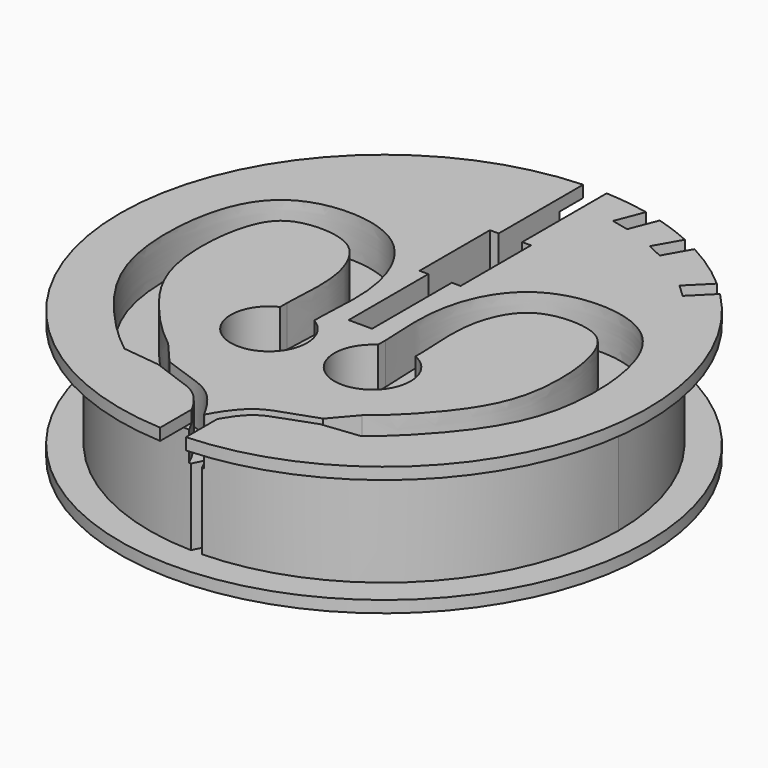
from build123d import *

# Parameters (mm, degrees)
F0_R           = 6.5
F1_DEPTH       = 22
F3_DEPTH       = 7
F5_DEPTH       = 6
F4_W           = 4
F4_H           = 17
F6_DEPTH       = 6
F7_DEPTH       = 9
F8_R           = 45
F8_R_2         = 40
F9_DEPTH       = 2
F10_START      = 20
F10_DEPTH      = 2
F11_DEPTH      = 4
F13_DEPTH      = 15
F13_DEPTH_BACK = 2
F14_W          = 3.2336955192
F14_H          = 3.9470121264
F15_DEPTH      = 2
F17_START      = 18
F17_DEPTH      = 4


# Not quite as in the source:
# - the dataset's text gives a spline's control points without its knots; the knots are read off the source's solid


with BuildPart() as f1:
    # F0 (on Top) → F1 (new body)
    with BuildSketch(Plane.XY):
        with BuildLine():
            ThreePointArc((0.9474656624, -39.9887772859), (28.6172904596, -27.9472840676), (40, 0))
            ThreePointArc((40, 0), (-27.9472840676, 28.6172904596), (-0.9474656624, -39.9887772859))
            add(Edge.make_bspline(
                [(0, -38.0722548049), (-0.3439047687, -38.7199985815), (-0.6597297626, -39.3669666276), (-0.9474656624, -39.9887772859)],
                knots=[0.8933636625, 0.8933636625, 0.8933636625, 0.8933636625, 1, 1, 1, 1], degree=3))
            add(Edge.make_bspline(
                [(0, -38.0722548049), (0.3439047687, -38.7199985815), (0.6597297626, -39.3669666276), (0.9474656624, -39.9887772859)],
                knots=[0.8933636625, 0.8933636625, 0.8933636625, 0.8933636625, 1, 1, 1, 1], degree=3))
        make_face()
        with Locations((-8.6927901772, -13.6614393054)):
            Circle(F0_R, mode=Mode.SUBTRACT)
        with Locations((8.9704493242, -13.6614393054)):
            Circle(F0_R, mode=Mode.SUBTRACT)
    extrude(amount=F1_DEPTH)

    # F2 (on face) → F3 (cut)
    with BuildSketch(Plane.XY.offset(22)):
        with BuildLine():
            Line((-11.4866509255, -6.2936628617), (-5.4897859509, -6.4875970689))
            add(Edge.make_bspline(
                [(-5.4897859509, -6.4875970689), (-5.4379960808, -4.8861423136), (-5.2594316262, -2.3960567313), (-5.21271863, 1.1661147071), (-5.3919407568, 3.966171195), (-5.9185254374, 6.8935002169), (-6.854038873, 9.8103742554), (-8.0244197776, 12.1448151724), (-9.2394760694, 13.8844575869), (-10.3025573556, 15.1020966662), (-11.5243351598, 16.2052705185), (-12.9191140784, 17.1606232553), (-14.3946005778, 17.9101133701), (-16.4368763853, 18.6735386839), (-19.0722321519, 19.2235783462), (-22.2281493374, 19.3375488673), (-24.7519752983, 19.0203587631), (-26.6553594717, 18.5206918318), (-28.4891702037, 17.8345146965), (-30.6169895374, 16.5861777721), (-32.3874729615, 14.8001880422), (-33.5420378244, 13.1039536454), (-34.2835644411, 11.7074846102), (-34.9043465841, 10.2008340024), (-35.5860681144, 8.0784891374), (-36.1962974623, 5.2321659425), (-36.5786674883, 1.6179124526), (-36.6190440844, -2.0722357876), (-36.3636264791, -5.1013980108), (-35.9747219859, -7.4398512499), (-35.4580158659, -9.6887320868), (-34.5932379657, -12.3018318431), (-33.2617334438, -15.1551375454), (-31.7045842952, -17.7556472269), (-30.2724053046, -19.7527908698), (-29.0788395713, -21.2722688411), (-27.8491903942, -22.7627774848), (-26.2467211141, -24.5683632891), (-23.5869366027, -27.2873636582), (-21.5286445413, -29.0857624272), (-20.1586929343, -30.1331636176)],
                knots=[0, 0, 0, 0, 0.0625, 0.09375, 0.125, 0.15625, 0.1875, 0.21875, 0.234375, 0.25, 0.265625, 0.28125, 0.296875, 0.3125, 0.34375, 0.375, 0.40625, 0.421875, 0.4375, 0.46875, 0.5, 0.515625, 0.53125, 0.546875, 0.5625, 0.59375, 0.625, 0.65625, 0.6875, 0.703125, 0.71875, 0.75, 0.78125, 0.8125, 0.84375, 0.859375, 0.875, 0.90625, 0.9375, 1, 1, 1, 1], degree=3))
            Line((-20.1586929343, -30.1331636176), (-16.5144508549, -25.3666659866))
            add(Edge.make_bspline(
                [(-11.4866509255, -6.2936628617), (-11.4582628575, -5.4158424255), (-11.3694789243, -3.707307233), (-11.2442598399, -1.2739253297), (-11.2217249783, 0.6576847954), (-11.2909792301, 2.1555003202), (-11.3951046961, 3.2596312313), (-11.5599404384, 4.3484374353), (-11.7949569978, 5.4365525911), (-12.100056325, 6.5030976742), (-12.5990453032, 7.8712270505), (-13.2319794554, 9.1203362077), (-13.9810727023, 10.1887494849), (-14.5951072186, 10.889894646), (-15.2595373513, 11.4865430576), (-15.97150147, 11.975035844), (-16.8044210088, 12.4016945204), (-18.0437162501, 12.8672967201), (-19.7854683017, 13.2380556024), (-21.6065908286, 13.3043531415), (-22.9949988463, 13.1866711855), (-23.9731162944, 13.0200835746), (-24.8514199077, 12.7876330323), (-25.8679172481, 12.4033835088), (-26.8953272178, 11.7912643881), (-27.7498799628, 10.9398607681), (-28.3866650169, 10.010963065), (-28.8365034761, 9.1692861425), (-29.2573618773, 8.1543752551), (-29.7633087928, 6.5871068241), (-30.2570042205, 4.3091059466), (-30.5797818082, 1.2755516731), (-30.6083344836, -1.3375574698), (-30.4846271103, -3.3824387204), (-30.3192794427, -4.8694397979), (-30.0837392894, -6.2819744334), (-29.6780655622, -8.0450529063), (-29.0044827772, -10.0809191806), (-27.958736191, -12.3252858014), (-26.6930020687, -14.4443827451), (-25.2271399739, -16.4914012395), (-23.5853711828, -18.5262777493), (-21.8535773868, -20.4784971841), (-19.4700703034, -22.9146854366), (-17.6631053951, -24.4884582261), (-16.5144508549, -25.3666659866)],
                knots=[0, 0, 0, 0, 0.03125, 0.0625, 0.09375, 0.109375, 0.125, 0.140625, 0.15625, 0.171875, 0.1875, 0.21875, 0.234375, 0.25, 0.265625, 0.28125, 0.296875, 0.3125, 0.34375, 0.375, 0.390625, 0.40625, 0.421875, 0.4375, 0.46875, 0.5, 0.515625, 0.53125, 0.546875, 0.5625, 0.59375, 0.625, 0.65625, 0.671875, 0.6875, 0.703125, 0.71875, 0.75, 0.78125, 0.8125, 0.84375, 0.875, 0.90625, 0.9375, 1, 1, 1, 1], degree=3))
        make_face()
        with BuildLine():
            Line((16.5129644521, -25.3766100658), (20.1572065315, -30.1431076968))
            add(Edge.make_bspline(
                [(5.4882995481, -6.4975411481), (5.4365096779, -4.8960863928), (5.2579452234, -2.4060008105), (5.2112322271, 1.1561706279), (5.390454354, 3.9562271158), (5.9170390346, 6.8835561377), (6.8525524702, 9.8004301762), (8.0229333747, 12.1348710933), (9.2379896666, 13.8745135078), (10.3010709528, 15.0921525871), (11.5228487569, 16.1953264394), (12.9176276756, 17.1506791761), (14.393114175, 17.900169291), (16.4353899825, 18.6635946047), (19.0707457491, 19.2136342671), (22.2266629346, 19.3276047881), (24.7504888954, 19.0104146839), (26.6538730688, 18.5107477526), (28.4876838008, 17.8245706173), (30.6155031345, 16.576233693), (32.3859865586, 14.7902439631), (33.5405514216, 13.0940095662), (34.2820780383, 11.6975405311), (34.9028601813, 10.1908899233), (35.5845817115, 8.0685450583), (36.1948110595, 5.2222218633), (36.5771810855, 1.6079683734), (36.6175576815, -2.0821798668), (36.3621400763, -5.11134209), (35.9732355831, -7.4497953291), (35.456529463, -9.698676166), (34.5917515628, -12.3117759223), (33.2602470409, -15.1650816246), (31.7030978923, -17.765591306), (30.2709189017, -19.762734949), (29.0773531685, -21.2822129203), (27.8477039913, -22.772721564), (26.2452347112, -24.5783073682), (23.5854501999, -27.2973077373), (21.5271581384, -29.0957065064), (20.1572065315, -30.1431076968)],
                knots=[0, 0, 0, 0, 0.0625, 0.09375, 0.125, 0.15625, 0.1875, 0.21875, 0.234375, 0.25, 0.265625, 0.28125, 0.296875, 0.3125, 0.34375, 0.375, 0.40625, 0.421875, 0.4375, 0.46875, 0.5, 0.515625, 0.53125, 0.546875, 0.5625, 0.59375, 0.625, 0.65625, 0.6875, 0.703125, 0.71875, 0.75, 0.78125, 0.8125, 0.84375, 0.859375, 0.875, 0.90625, 0.9375, 1, 1, 1, 1], degree=3))
            Line((5.4882995481, -6.4975411481), (5.4882995481, -8.172848144))
            ThreePointArc((5.4882995481, -8.172848144), (8.4247356636, -7.1843877693), (11.4851645226, -7.6675918373))
            Line((11.4851645226, -7.6675918373), (11.4851645226, -6.3036069409))
            add(Edge.make_bspline(
                [(11.4851645226, -6.3036069409), (11.4567764547, -5.4257865047), (11.3679925215, -3.7172513122), (11.2427734371, -1.2838694089), (11.2202385755, 0.6477407162), (11.2894928273, 2.1455562411), (11.3936182933, 3.2496871522), (11.5584540356, 4.3384933561), (11.793470595, 5.4266085119), (12.0985699221, 6.493153595), (12.5975589004, 7.8612829714), (13.2304930526, 9.1103921285), (13.9795862995, 10.1788054057), (14.5936208158, 10.8799505668), (15.2580509484, 11.4765989785), (15.9700150672, 11.9650917649), (16.802934606, 12.3917504412), (18.0422298473, 12.857352641), (19.7839818989, 13.2281115232), (21.6051044257, 13.2944090623), (22.9935124434, 13.1767271063), (23.9716298916, 13.0101394954), (24.8499335049, 12.7776889531), (25.8664308452, 12.3934394297), (26.893840815, 11.781320309), (27.74839356, 10.9299166889), (28.3851786141, 10.0010189859), (28.8350170732, 9.1593420634), (29.2558754745, 8.1444311759), (29.76182239, 6.5771627449), (30.2555178176, 4.2991618675), (30.5782954054, 1.2656075939), (30.6068480808, -1.347501549), (30.4831407075, -3.3923827996), (30.3177930399, -4.8793838771), (30.0822528866, -6.2919185126), (29.6765791594, -8.0549969855), (29.0029963744, -10.0908632598), (27.9572497882, -12.3352298806), (26.6915156658, -14.4543268243), (25.2256535711, -16.5013453187), (23.5838847799, -18.5362218284), (21.8520909839, -20.4884412632), (19.4685839006, -22.9246295158), (17.6616189923, -24.4984023052), (16.5129644521, -25.3766100658)],
                knots=[0, 0, 0, 0, 0.03125, 0.0625, 0.09375, 0.109375, 0.125, 0.140625, 0.15625, 0.171875, 0.1875, 0.21875, 0.234375, 0.25, 0.265625, 0.28125, 0.296875, 0.3125, 0.34375, 0.375, 0.390625, 0.40625, 0.421875, 0.4375, 0.46875, 0.5, 0.515625, 0.53125, 0.546875, 0.5625, 0.59375, 0.625, 0.65625, 0.671875, 0.6875, 0.703125, 0.71875, 0.75, 0.78125, 0.8125, 0.84375, 0.875, 0.90625, 0.9375, 1, 1, 1, 1], degree=3))
        make_face()
        with BuildLine():
            Line((-5.4897859509, -8.0054014761), (-5.4897859509, -6.4875970689))
            Line((-5.4897859509, -6.4875970689), (-11.4866509255, -6.2936628617))
            Line((-11.4866509255, -6.2936628617), (-11.4866509255, -7.792509069))
            ThreePointArc((-11.4866509255, -7.792509069), (-8.4621814379, -7.1655313927), (-5.4897859509, -8.0054014761))
        make_face()
        with BuildLine():
            Line((-5.4897859509, -8.2850931604), (-5.4897859509, -8.0054014761))
            ThreePointArc((-5.4897859509, -8.0054014761), (-8.4621814379, -7.1655313927), (-11.4866509255, -7.792509069))
            Line((-11.4866509255, -7.792509069), (-11.4866509255, -8.0895419435))
            Line((-11.4866509255, -8.0895419435), (-5.4897859509, -8.2850931604))
        make_face()
        with BuildLine():
            Line((-13.1143264077, -29.3359424549), (-13.7970289215, -30.8739412576))
            add(Edge.make_bspline(
                [(-13.7970289215, -30.8739412576), (-12.5260111469, -31.3816306977), (-10.266053309, -32.1850470743), (-8.1581038581, -32.8766105177), (-6.8097358347, -33.4182948064), (-5.9513697948, -33.8527961491), (-5.323719903, -34.2737444381), (-4.8436087243, -34.6763658921), (-4.3647349622, -35.13515786), (-3.7779019908, -35.8008156001), (-3.1027106535, -36.7184324149), (-2.4647104355, -37.7223140251), (-1.8467043429, -38.8200104181), (-1.4615503002, -39.5814813981), (-1.2687707391, -39.9798726963)],
                knots=[0.1305954115, 0.1305954115, 0.1305954115, 0.1305954115, 0.25, 0.375, 0.4375, 0.5, 0.5625, 0.59375, 0.625, 0.6875, 0.75, 0.8125, 0.875, 0.9445236509, 0.9445236509, 0.9445236509, 0.9445236509], degree=3))
            ThreePointArc((-1.2687707391, -39.9798726963), (-1.1081271451, -39.9846477317), (-0.9474656624, -39.9887772859))
            add(Edge.make_bspline(
                [(-0.0803490442, -38.2245407637), (-0.3932414238, -38.8212637523), (-0.6822827282, -39.415704635), (-0.9474656624, -39.9887772859)],
                knots=[0.9017219024, 0.9017219024, 0.9017219024, 0.9017219024, 1, 1, 1, 1], degree=3))
            add(Edge.make_bspline(
                [(-13.1143264077, -29.3359424549), (-11.9194556955, -29.7996228015), (-9.7599118859, -30.5474299547), (-7.6478529152, -31.2193926834), (-6.133292009, -31.8104744748), (-5.0776722344, -32.3308818456), (-4.0856391538, -32.9823429694), (-3.1609110891, -33.8033335861), (-2.3197029068, -34.7451125479), (-1.2878110507, -36.1251687047), (-0.5665560799, -37.3256310433), (-0.117832094, -38.1546758024), (-0.0803490442, -38.2245407637)],
                knots=[0.1336233385, 0.1336233385, 0.1336233385, 0.1336233385, 0.25, 0.375, 0.4375, 0.5, 0.5625, 0.625, 0.6875, 0.75, 0.875, 0.886501703, 0.886501703, 0.886501703, 0.886501703], degree=3))
        make_face()
        Polygon((13.1128400049, -29.3458865341), (13.7939090688, -30.8604739264), (20.1572065315, -30.1431076968), (16.5129644521, -25.3766100658), align=None)
        Polygon((-16.5144508549, -25.3666659866), (-20.1586929343, -30.1331636176), (-13.7970289215, -30.8739412576), (-13.1143264077, -29.3359424549), align=None)
        with BuildLine():
            ThreePointArc((0.9474656624, -39.9887772859), (1.1049034783, -39.9847369418), (1.2623241662, -39.9800767595))
            add(Edge.make_bspline(
                [(13.7939090688, -30.8604739264), (12.5246046617, -31.3673755436), (10.266128995, -32.1702409999), (8.1590553393, -32.8615171177), (6.8106873159, -33.4032014064), (5.952321276, -33.8377027491), (5.3246713842, -34.2586510381), (4.8445602054, -34.6612724921), (4.3656864434, -35.12006446), (3.778853472, -35.7857222001), (3.1036621346, -36.7033390149), (2.4656619167, -37.7072206251), (1.8448284848, -38.8099389106), (1.4573109135, -39.5766544611), (1.2623241662, -39.9800767595)],
                knots=[0.1307229219, 0.1307229219, 0.1307229219, 0.1307229219, 0.25, 0.375, 0.4375, 0.5, 0.5625, 0.59375, 0.625, 0.6875, 0.75, 0.8125, 0.875, 0.9454135844, 0.9454135844, 0.9454135844, 0.9454135844], degree=3))
            Line((13.7939090688, -30.8604739264), (13.1128400049, -29.3458865341))
            add(Edge.make_bspline(
                [(13.1128400049, -29.3458865341), (11.9179692927, -29.8095668807), (9.758425483, -30.5573740339), (7.6463665124, -31.2293367626), (6.1318056062, -31.8204185539), (5.0761858316, -32.3408259248), (4.084152751, -32.9922870485), (3.1594246863, -33.8132776653), (2.318216504, -34.7550566271), (1.2863246479, -36.1351127839), (0.5663256909, -37.3334846033), (0.1186244068, -38.1604104004), (0.0822516327, -38.2281697586)],
                knots=[0.1336233385, 0.1336233385, 0.1336233385, 0.1336233385, 0.25, 0.375, 0.4375, 0.5, 0.5625, 0.625, 0.6875, 0.75, 0.875, 0.8861551558, 0.8861551558, 0.8861551558, 0.8861551558], degree=3))
            add(Edge.make_bspline(
                [(0.0822516327, -38.2281697586), (0.3944132124, -38.8236737608), (0.682820306, -39.4168663655), (0.9474656624, -39.9887772859)],
                knots=[0.9019211313, 0.9019211313, 0.9019211313, 0.9019211313, 1, 1, 1, 1], degree=3))
        make_face()
    extrude(amount=-F3_DEPTH, mode=Mode.SUBTRACT)

    # F4 (on face) → F5 (cut)
    with BuildSketch(Plane.XY.offset(22)):
        with BuildLine():
            Line((2, 39.9499687109), (2, 51.9499687109))
            Line((2, 51.9499687109), (-2, 51.9499687109))
            Line((-2, 51.9499687109), (-2, 39.9499687109))
            ThreePointArc((-2, 39.9499687109), (0, 40), (2, 39.9499687109))
        make_face()
        with BuildLine():
            Line((2, 26.9499687109), (2, 39.9499687109))
            ThreePointArc((2, 39.9499687109), (0, 40), (-2, 39.9499687109))
            Line((-2, 39.9499687109), (-2, 26.9499687109))
            Line((-2, 26.9499687109), (2, 26.9499687109))
        make_face()
    extrude(amount=-F5_DEPTH, mode=Mode.SUBTRACT)

    # F4 (on face) → F6 (cut)
    with BuildSketch(Plane.XY.offset(22)):
        with Locations((0, 3.4499687109)):
            Rectangle(F4_W, F4_H)
    extrude(amount=-F6_DEPTH, mode=Mode.SUBTRACT)

    # F4 (on face) → F7 (cut)
    with BuildSketch(Plane.XY.offset(22)):
        Polygon((3.5, 26.9499687109), (2, 26.9499687109), (-2, 26.9499687109), (-3.5, 26.9499687109), (-3.5, 11.9499687109), (-2, 11.9499687109), (2, 11.9499687109), (3.5, 11.9499687109), align=None)
    extrude(amount=-F7_DEPTH, mode=Mode.SUBTRACT)

    # F8 (on Top) → F9 (join)
    with BuildSketch(Plane.XY):
        Circle(F8_R)
        Circle(F8_R_2, mode=Mode.SUBTRACT)
    extrude(amount=F9_DEPTH)

    # F8 (on Top) → F10 (join)
    with BuildSketch(Plane.XY.offset(F10_START)):
        Circle(F8_R)
        Circle(F8_R_2, mode=Mode.SUBTRACT)
    extrude(amount=F10_DEPTH)

    # F4 (on face) → F11 (cut)
    with BuildSketch(Plane.XY.offset(22)):
        with BuildLine():
            Line((2, 39.9499687109), (2, 51.9499687109))
            Line((2, 51.9499687109), (-2, 51.9499687109))
            Line((-2, 51.9499687109), (-2, 39.9499687109))
            ThreePointArc((-2, 39.9499687109), (0, 40), (2, 39.9499687109))
        make_face()
    extrude(amount=-F11_DEPTH, mode=Mode.SUBTRACT)

    # F12 (on face) → F13 (cut, two sides)
    with BuildSketch(Plane.XY.offset(22)) as f13_sk:
        with BuildLine():
            Line((2.1751223091, -45.7168594003), (2.1751223091, -44.9474008474))
            ThreePointArc((2.1751223092, -44.9474008474), (-0.0215743842, -44.9999948283), (-2.2182196374, -44.9452945439))
            Line((-2.2182196374, -44.9452945439), (-2.2182196374, -45.7168594003))
            Line((-2.2182196374, -45.7168594003), (2.1751223091, -45.7168594003))
        make_face()
        with BuildLine():
            Line((2.1751223091, -44.9474008474), (2.1751223091, -38.228169755))
            add(Edge.make_bspline(
                [(2.1751223091, -38.228169755), (2.0740297915, -38.407010603), (1.755389532, -38.9868966566), (1.4573109135, -39.5766544611), (1.2623241662, -39.9800767595)],
                knots=[0.8431764201, 0.8431764201, 0.8431764201, 0.8431764201, 0.875, 0.9454135844, 0.9454135844, 0.9454135844, 0.9454135844], degree=3))
            ThreePointArc((1.2623241662, -39.9800767595), (-0.0032249009, -39.99999987), (-1.2687707391, -39.9798726963))
            add(Edge.make_bspline(
                [(-2.1827093746, -38.228169755), (-2.0786618127, -38.411946344), (-1.7598241179, -38.9917774588), (-1.4615503002, -39.5814813981), (-1.2687707391, -39.9798726963)],
                knots=[0.8422809272, 0.8422809272, 0.8422809272, 0.8422809272, 0.875, 0.9445236509, 0.9445236509, 0.9445236509, 0.9445236509], degree=3))
            Line((-2.1827093746, -38.228169755), (-2.2182196374, -38.228169755))
            Line((-2.2182196374, -38.228169755), (-2.2182196374, -44.9452945439))
            ThreePointArc((-2.2182196374, -44.9452945439), (-0.0215743842, -44.9999948283), (2.1751223092, -44.9474008474))
        make_face()
    extrude(amount=F13_DEPTH, mode=Mode.SUBTRACT)
    extrude(f13_sk.sketch, amount=-F13_DEPTH_BACK, mode=Mode.SUBTRACT)

    # F14 (on Top) → F15 (join)
    with BuildSketch(Plane.XY):
        with Locations((-0.0080559985, -39.2427109182)):
            Rectangle(F14_W, F14_H)
    extrude(amount=F15_DEPTH)

    # F16 (on face) → F17 (cut)
    with BuildSketch(Plane.XY.offset(2).offset(F17_START)):
        Polygon((7.6347516803, 39.2646223308), (10.5850033616, 38.5740548016), (12.8356672982, 44.3638138473), (9.9028458584, 45.0992201003), align=None)
        Polygon((16.0097401568, 36.6563530662), (18.7179382503, 35.3502303763), (21.7398184516, 40.6750121187), (19.0426836581, 42.0006291809), align=None)
        Polygon((26.183301022, 30.239622147), (28.3773642629, 28.1908708182), (32.6035102987, 32.407085155), (30.4192533119, 34.4656196926), align=None)
    extrude(amount=F17_DEPTH, mode=Mode.SUBTRACT)


solid = f1.part
